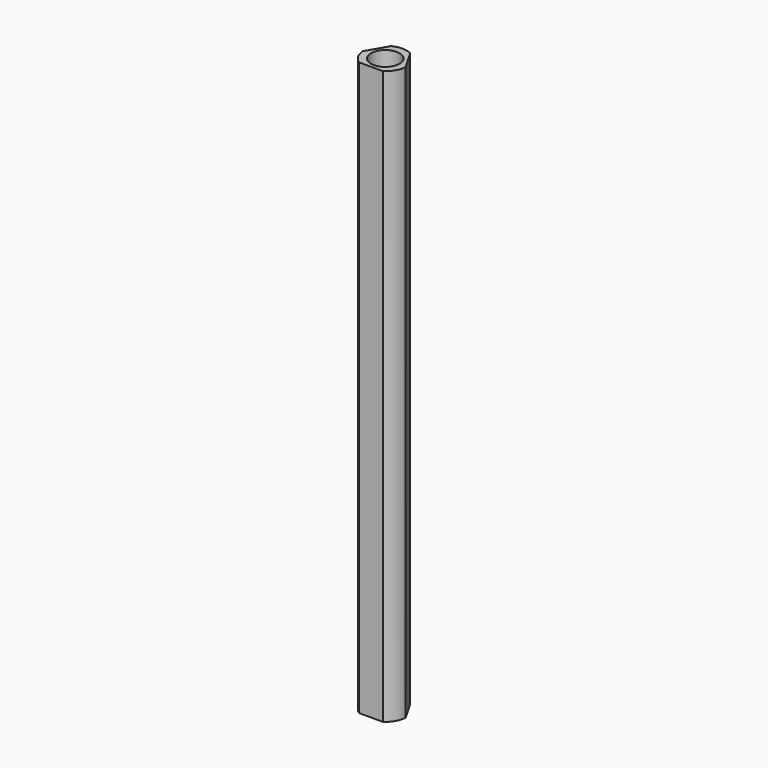
from build123d import *

# Parameters (mm, degrees)
F0_R            = 9
F0_R_2          = 6
F1_DEPTH        = 240
F3_W            = 18
F3_H            = 240
F4_DEPTH        = 1.5
F4_COPIES_COUNT = 3


# Not quite as in the source:
# - a pattern or mirror of a feature is missing from the dataset's text; its kind, count and spacing are read off the source's solid


with BuildPart() as f1:
    # F0 (on Top) → F1 (new body)
    with BuildSketch(Plane.XY):
        Circle(F0_R)
        Circle(F0_R_2, mode=Mode.SUBTRACT)
    extrude(amount=F1_DEPTH)

    # F3 (on offset) → F4 (cut)
    with BuildSketch(Plane.XZ.offset(9)):
        with Locations((0, 120)):
            Rectangle(F3_W, F3_H)
    f4 = extrude(amount=-F4_DEPTH, mode=Mode.SUBTRACT)

    # F4_copies: F4 ×3 about axis
    f4_copies_axis = Axis((0, 0, 0), (0, 0, 1))
    for i in range(1, F4_COPIES_COUNT):
        add(f4.rotate(f4_copies_axis, i * 360 / F4_COPIES_COUNT), mode=Mode.SUBTRACT)


solid = f1.part
